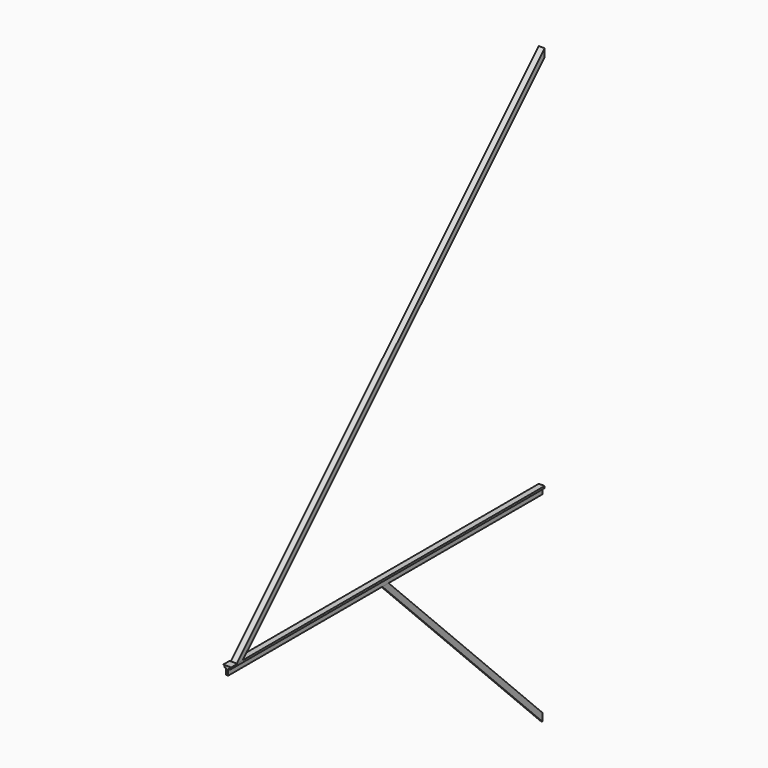
from build123d import *

# Parameters (mm, degrees)
F1_DEPTH = 500
F3_DEPTH = 7.5
F5_DEPTH = 2.5
F6_W     = 1.25
F6_H     = 10
F6_W_2   = 7.5
F7_DEPTH = 0.5


with BuildPart() as f1:
    # F0 (on Front) → F1 (new body)
    with BuildSketch(Plane.XZ):
        Polygon((-1.25, 3.75), (-1.25, -3.75), (1.25, -3.75), (1.25, 3.75), (3.75, 3.75), (3.75, 6.25), (-3.75, 6.25), (-3.75, 3.75), align=None)
    extrude(amount=F1_DEPTH)

    # F6 (on face) → F7 (join)
    with BuildSketch(Plane.XY.offset(6.25)):
        with Locations((4.375, -495)):
            Rectangle(F6_W, F6_H)
        with Locations((0, -495)):
            Rectangle(F6_W_2, F6_H)
        with Locations((-4.375, -495)):
            Rectangle(F6_W, F6_H)
    extrude(amount=F7_DEPTH)


with BuildPart() as f3:
    # F2 (on face) → F3 (new body)
    with BuildSketch(Plane(origin=(-3.75, 0, 0), x_dir=(0, -1, 0), z_dir=(-1, 0, 0))):
        Polygon((490, 6.25), (0, 496.25), (0, 486.25), (480, 6.25), align=None)
    extrude(amount=-F3_DEPTH)


with BuildPart() as f5:
    # F4 (on face) → F5 (new body)
    with BuildSketch(Plane(origin=(-1.25, 0, 0), x_dir=(0, -1, 0), z_dir=(-1, 0, 0))):
        Polygon((245, -3.75), (0, -248.75), (0, -258.75), (255, -3.75), align=None)
    extrude(amount=-F5_DEPTH)


solid = Compound([f1.part, f3.part, f5.part])
